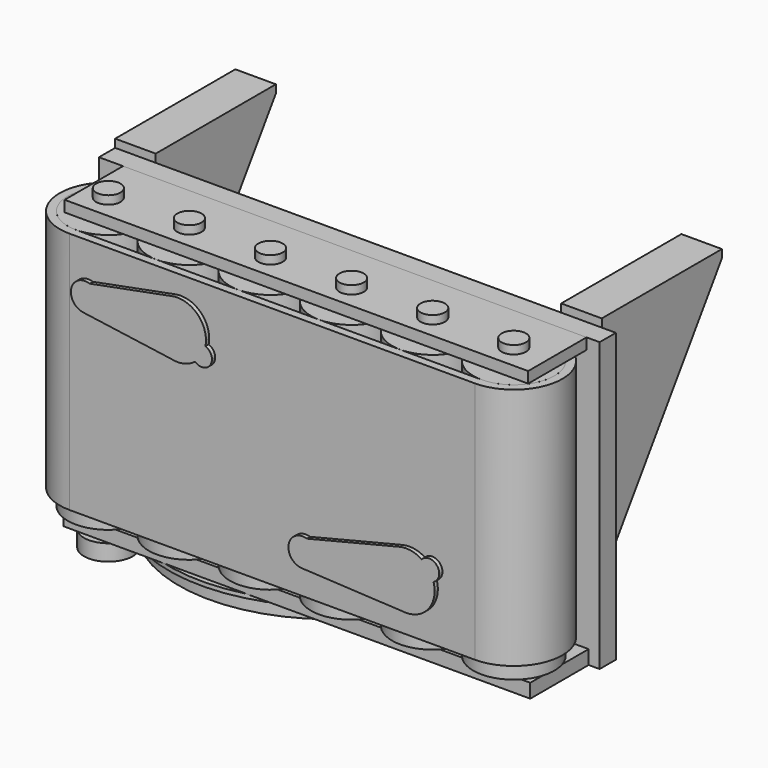
from build123d import *

# Parameters (mm, degrees)
F0_R      = 50
F1_DEPTH  = 300
F2_DEPTH  = 20
F3_R      = 15
F4_DEPTH  = 25
F5_DEPTH  = 345
F6_R      = 30
F7_DEPTH  = 20
F9_DEPTH  = 300
F10_W     = 617.369171232
F10_H     = 354.843031615
F11_DEPTH = 25
F12_W     = 571.5557485819
F12_H     = 13.6696398258
F13_DEPTH = 90
F14_W     = 575.6089426577
F14_H     = 17.266811803
F15_DEPTH = 90
F17_DEPTH = 50
F19_W     = 290.3259024024
F19_H     = 23.030102253
F20_DEPTH = 174
F22_DEPTH = 290.3259024024
F23_R     = 187.1632519627
F24_DEPTH = 20
F25_R     = 15
F26_DEPTH = 70
F28_DEPTH = 5
F29_R     = 199.2283933236
F30_DEPTH = 5
F31_R     = 2.5
F32_DEPTH = 2
F33_COUNT = 18
F34_W     = 50
F34_H     = 185.2015340328
F35_DEPTH = 10
F36_W     = 50
F36_H     = 185.2015340328
F37_DEPTH = 10
F38_R     = 10
F39_DEPTH = 60
F40_W     = 67.3258155584
F40_H     = 104.313146323
F41_DEPTH = 139


with BuildPart() as f1:
    # F0 (on Top) → F1 (new body)
    with BuildSketch(Plane.XY):
        Circle(F0_R)
    extrude(amount=F1_DEPTH)


with BuildPart() as f1b:
    # F0 (on Top) → F1, piece 2 (new body)
    with BuildSketch(Plane.XY):
        with BuildLine():
            ThreePointArc((550, 0), (500, 50), (450, 0))
            ThreePointArc((450, 0), (500, -50), (550, 0))
        make_face()
    extrude(amount=F1_DEPTH)


with BuildPart() as f1c:
    # F0 (on Top) → F1, piece 3 (new body)
    with BuildSketch(Plane.XY):
        with BuildLine():
            ThreePointArc((450, 0), (400, 50), (350, 0))
            ThreePointArc((350, 0), (400, -50), (450, 0))
        make_face()
    extrude(amount=F1_DEPTH)


with BuildPart() as f1d:
    # F0 (on Top) → F1, piece 4 (new body)
    with BuildSketch(Plane.XY):
        with BuildLine():
            ThreePointArc((350, 0), (300, 50), (250, 0))
            ThreePointArc((250, 0), (300, -50), (350, 0))
        make_face()
    extrude(amount=F1_DEPTH)


with BuildPart() as f1e:
    # F0 (on Top) → F1, piece 5 (new body)
    with BuildSketch(Plane.XY):
        with BuildLine():
            ThreePointArc((250, 0), (200, 50), (150, 0))
            ThreePointArc((150, 0), (200, -50), (250, 0))
        make_face()
    extrude(amount=F1_DEPTH)


with BuildPart() as f1f:
    # F0 (on Top) → F1, piece 6 (new body)
    with BuildSketch(Plane.XY):
        with BuildLine():
            ThreePointArc((150, 0), (100, 50), (50, 0))
            ThreePointArc((50, 0), (100, -50), (150, 0))
        make_face()
    extrude(amount=F1_DEPTH)


with BuildPart() as f2:
    # F0 (on Top) → F2 (new body)
    with BuildSketch(Plane.XY):
        Circle(F0_R)
    extrude(amount=-F2_DEPTH)


with BuildPart() as f2b:
    # F0 (on Top) → F2, piece 2 (new body)
    with BuildSketch(Plane.XY):
        with BuildLine():
            ThreePointArc((550, 0), (500, 50), (450, 0))
            ThreePointArc((450, 0), (500, -50), (550, 0))
        make_face()
    extrude(amount=-F2_DEPTH)


with BuildPart() as f2c:
    # F0 (on Top) → F2, piece 3 (new body)
    with BuildSketch(Plane.XY):
        with BuildLine():
            ThreePointArc((450, 0), (400, 50), (350, 0))
            ThreePointArc((350, 0), (400, -50), (450, 0))
        make_face()
    extrude(amount=-F2_DEPTH)


with BuildPart() as f2d:
    # F0 (on Top) → F2, piece 4 (new body)
    with BuildSketch(Plane.XY):
        with BuildLine():
            ThreePointArc((350, 0), (300, 50), (250, 0))
            ThreePointArc((250, 0), (300, -50), (350, 0))
        make_face()
    extrude(amount=-F2_DEPTH)


with BuildPart() as f2e:
    # F0 (on Top) → F2, piece 5 (new body)
    with BuildSketch(Plane.XY):
        with BuildLine():
            ThreePointArc((250, 0), (200, 50), (150, 0))
            ThreePointArc((150, 0), (200, -50), (250, 0))
        make_face()
    extrude(amount=-F2_DEPTH)


with BuildPart() as f2f:
    # F0 (on Top) → F2, piece 6 (new body)
    with BuildSketch(Plane.XY):
        with BuildLine():
            ThreePointArc((150, 0), (100, 50), (50, 0))
            ThreePointArc((50, 0), (100, -50), (150, 0))
        make_face()
    extrude(amount=-F2_DEPTH)


with BuildPart() as f4:
    # F3 (on face) → F4 (new body)
    with BuildSketch(Plane(origin=(0, 0, -20), x_dir=(1, 0, 0), z_dir=(0, 0, -1))):
        Circle(F3_R)
    extrude(amount=F4_DEPTH)


with BuildPart() as f4b:
    # F3 (on face) → F4, piece 2 (new body)
    with BuildSketch(Plane(origin=(0, 0, -20), x_dir=(1, 0, 0), z_dir=(0, 0, -1))):
        with Locations((100, 0)):
            Circle(F3_R)
    extrude(amount=F4_DEPTH)


with BuildPart() as f4c:
    # F3 (on face) → F4, piece 3 (new body)
    with BuildSketch(Plane(origin=(0, 0, -20), x_dir=(1, 0, 0), z_dir=(0, 0, -1))):
        with Locations((200, 0)):
            Circle(F3_R)
    extrude(amount=F4_DEPTH)


with BuildPart() as f4d:
    # F3 (on face) → F4, piece 4 (new body)
    with BuildSketch(Plane(origin=(0, 0, -20), x_dir=(1, 0, 0), z_dir=(0, 0, -1))):
        with Locations((300, 0)):
            Circle(F3_R)
    extrude(amount=F4_DEPTH)


with BuildPart() as f4e:
    # F3 (on face) → F4, piece 5 (new body)
    with BuildSketch(Plane(origin=(0, 0, -20), x_dir=(1, 0, 0), z_dir=(0, 0, -1))):
        with Locations((400, 0)):
            Circle(F3_R)
    extrude(amount=F4_DEPTH)


with BuildPart() as f4f:
    # F3 (on face) → F4, piece 6 (new body)
    with BuildSketch(Plane(origin=(0, 0, -20), x_dir=(1, 0, 0), z_dir=(0, 0, -1))):
        with Locations((500, 0)):
            Circle(F3_R)
    extrude(amount=F4_DEPTH)


with BuildPart() as f5:
    # F3 (on face) → F5 (new body)
    with BuildSketch(Plane(origin=(0, 0, -20), x_dir=(1, 0, 0), z_dir=(0, 0, -1))):
        Circle(F3_R)
    extrude(amount=-F5_DEPTH)


with BuildPart() as f5b:
    # F3 (on face) → F5, piece 2 (new body)
    with BuildSketch(Plane(origin=(0, 0, -20), x_dir=(1, 0, 0), z_dir=(0, 0, -1))):
        with Locations((100, 0)):
            Circle(F3_R)
    extrude(amount=-F5_DEPTH)


with BuildPart() as f5c:
    # F3 (on face) → F5, piece 3 (new body)
    with BuildSketch(Plane(origin=(0, 0, -20), x_dir=(1, 0, 0), z_dir=(0, 0, -1))):
        with Locations((200, 0)):
            Circle(F3_R)
    extrude(amount=-F5_DEPTH)


with BuildPart() as f5d:
    # F3 (on face) → F5, piece 4 (new body)
    with BuildSketch(Plane(origin=(0, 0, -20), x_dir=(1, 0, 0), z_dir=(0, 0, -1))):
        with Locations((300, 0)):
            Circle(F3_R)
    extrude(amount=-F5_DEPTH)


with BuildPart() as f5e:
    # F3 (on face) → F5, piece 5 (new body)
    with BuildSketch(Plane(origin=(0, 0, -20), x_dir=(1, 0, 0), z_dir=(0, 0, -1))):
        with Locations((400, 0)):
            Circle(F3_R)
    extrude(amount=-F5_DEPTH)


with BuildPart() as f5f:
    # F3 (on face) → F5, piece 6 (new body)
    with BuildSketch(Plane(origin=(0, 0, -20), x_dir=(1, 0, 0), z_dir=(0, 0, -1))):
        with Locations((500, 0)):
            Circle(F3_R)
    extrude(amount=-F5_DEPTH)


with BuildPart() as f7:
    # F6 (on face) → F7 (new body)
    with BuildSketch(Plane(origin=(0, 0, -45), x_dir=(1, 0, 0), z_dir=(0, 0, -1))):
        Circle(F6_R)
    extrude(amount=F7_DEPTH)


with BuildPart() as f9:
    # F8 (on face) → F9 (new body)
    with BuildSketch(Plane.XY.offset(300)):
        with BuildLine():
            Line((500, 60), (0, 60))
            ThreePointArc((0, 60), (-60, 0), (0, -60))
            Line((0, -60), (500, -60))
            ThreePointArc((500, -60), (560, 0), (500, 60))
        make_face()
        with BuildLine():
            ThreePointArc((0, -50), (-50, 0), (0, 50))
            Line((0, 50), (500, 50))
            ThreePointArc((500, 50), (550, 0), (500, -50))
            Line((500, -50), (0, -50))
        make_face(mode=Mode.SUBTRACT)
    extrude(amount=-F9_DEPTH)


with BuildPart() as f11:
    # F10 (on face) → F11 (new body)
    with BuildSketch(Plane(origin=(0, 60, 0), x_dir=(-1, 0, 0), z_dir=(0, 1, 0))):
        with Locations((-249.1421122104, 137.3082045466)):
            Rectangle(F10_W, F10_H)
    extrude(amount=F11_DEPTH)

    # F19 (on face) → F20 (join)
    with BuildSketch(Plane(origin=(0, 85, 0), x_dir=(-1, 0, 0), z_dir=(0, 1, 0))):
        with Locations((-225.6603725255, -28.5982601345)):
            Rectangle(F19_W, F19_H)
    extrude(amount=F20_DEPTH)

    # F21 (on face) → F22 (join, through all)
    with BuildSketch(Plane(origin=(80.4974213243, 0, 0), x_dir=(0, -1, 0), z_dir=(-1, 0, 0))):
        Polygon((-85, 129.8807710409), (-259, -17.083209008), (-85, -17.083209008), align=None)
    extrude(amount=-F22_DEPTH)

    # F40 (on face) → F41 (cut)
    with BuildSketch(Plane(origin=(0, 259, 0), x_dir=(-1, 0, 0), z_dir=(0, 1, 0))):
        with Locations((-145.5224826932, 35.0733641535)):
            Rectangle(F40_W, F40_H)
    extrude(amount=-F41_DEPTH, mode=Mode.SUBTRACT)


with BuildPart() as f13:
    # F12 (on face) → F13 (new body)
    with BuildSketch(Plane.XZ.offset(-60)):
        with Locations((255.916647613, 307.8949004412)):
            Rectangle(F12_W, F12_H)
    extrude(amount=F13_DEPTH)


with BuildPart() as f15:
    # F14 (on face) → F15 (new body)
    with BuildSketch(Plane.XZ.offset(-60)):
        with Locations((256.457997486, -31.4799053594)):
            Rectangle(F14_W, F14_H)
    extrude(amount=F15_DEPTH)


with BuildPart() as f17:
    # F16 (on face) → F17 (new body)
    with BuildSketch(Plane(origin=(-59.5424734056, 0, 0), x_dir=(0, -1, 0), z_dir=(-1, 0, 0))):
        Polygon((-270.2015340328, 314.7297203541), (-85, 41.2701405585), (-85, 314.7297203541), align=None)
    extrude(amount=-F17_DEPTH)


with BuildPart() as f18_1:
    # F18: copy of F17
    add(f17.part.moved(Location((550, 0, 0))))

    # F34 (on face) → F35 (join)
    with BuildSketch(Plane.XY.offset(314.7297203541)):
        with Locations((515.4575265944, 177.6007670164)):
            Rectangle(F34_W, F34_H)
    extrude(amount=F35_DEPTH)


with BuildPart() as f24:
    # F23 (on face) → F24 (new body)
    with BuildSketch(Plane(origin=(0, 0, -65), x_dir=(1, 0, 0), z_dir=(0, 0, -1))):
        with Locations((143.8672691584, -162.6717150211)):
            Circle(F23_R)
    extrude(amount=-F24_DEPTH)

    # F25 (on face) → F26 (join)
    with BuildSketch(Plane(origin=(0, 0, -65), x_dir=(1, 0, 0), z_dir=(0, 0, -1))):
        with Locations((273.0099856853, -139.8850679398)):
            Circle(F25_R)
    extrude(amount=F26_DEPTH)

    # F38 (on face) → F39 (join)
    with BuildSketch(Plane(origin=(0, 0, -65), x_dir=(1, 0, 0), z_dir=(0, 0, -1))):
        with Locations((143.8672691584, -162.6717150211)):
            Circle(F38_R)
    extrude(amount=-F39_DEPTH)


with BuildPart() as f28:
    # F27 (on face) → F28 (new body)
    with BuildSketch(Plane.XZ.offset(60)):
        with BuildLine():
            ThreePointArc((290.6598971339, 33.2716024848), (303.6093206658, 38.0614510744), (309.0558983607, 50.7486497697))
            ThreePointArc((309.0558983607, 50.7486497697), (305.6933150557, 61.0628850392), (296.8977898815, 67.4134088433))
            ThreePointArc((296.8977898815, 67.4134088433), (274.3408694475, 53.8939286949), (290.6598971339, 33.2716024848))
        make_face()
        with BuildLine():
            ThreePointArc((296.8977898815, 67.4134088433), (305.6933150557, 61.0628850392), (309.0558983607, 50.7486497697))
            ThreePointArc((309.0558983607, 50.7486497697), (303.6093206658, 38.0614510744), (290.6598971339, 33.2716024848))
            Line((290.6598971339, 33.2716024848), (415.7583559022, 26.8581408344))
            ThreePointArc((415.7583559022, 26.8581408344), (384.4237307256, 59.2215727659), (410.9251114785, 95.648585813))
            Line((410.9251114785, 95.648585813), (296.8977898815, 67.4134088433))
        make_face()
        with BuildLine():
            Line((419.3376600868, 26.6746395319), (410.9251114785, 95.648585813))
            ThreePointArc((410.9251114785, 95.648585813), (384.4237307256, 59.2215727659), (415.7583559022, 26.8581408344))
            Line((415.7583559022, 26.8581408344), (419.3376600868, 26.6746395319))
        make_face()
        with BuildLine():
            ThreePointArc((438.4152543286, 91.0182146028), (425.1510828288, 96.1884645303), (410.9251114785, 95.648585813))
            Line((410.9251114785, 95.648585813), (419.3376600868, 26.6746395319))
            ThreePointArc((419.3376600868, 26.6746395319), (444.0863974283, 36.9259021903), (454.3376600868, 61.6746395319))
            ThreePointArc((454.3376600868, 61.6746395319), (454.0044818165, 66.4924680017), (453.011290306, 71.2185709997))
            ThreePointArc((453.011290306, 71.2185709997), (437.4484346974, 75.0256635752), (438.4152543286, 91.0182146028))
        make_face()
        with BuildLine():
            Line((419.3376600868, 26.6746395319), (415.7583559022, 26.8581408344))
            ThreePointArc((415.7583559022, 26.8581408344), (417.5456576332, 26.7205449619), (419.3376600868, 26.6746395319))
        make_face()
        with BuildLine():
            ThreePointArc((460.0099761477, 82.4428991548), (452.1233251081, 94.060429502), (438.4152543286, 91.0182146028))
            ThreePointArc((438.4152543286, 91.0182146028), (447.5099761477, 82.4428991548), (453.011290306, 71.2185709997))
            ThreePointArc((453.011290306, 71.2185709997), (458.116965046, 75.8291417877), (460.0099761477, 82.4428991548))
        make_face()
        with BuildLine():
            ThreePointArc((453.011290306, 71.2185709997), (447.5099761477, 82.4428991548), (438.4152543286, 91.0182146028))
            ThreePointArc((438.4152543286, 91.0182146028), (437.4484346974, 75.0256635752), (453.011290306, 71.2185709997))
        make_face()
    extrude(amount=F28_DEPTH)


with BuildPart() as f28b:
    # F27 (on face) → F28, piece 2 (new body)
    with BuildSketch(Plane.XZ.offset(60)):
        with BuildLine():
            ThreePointArc((158.9437698468, 214.6585216105), (172.3725190643, 212.5876755669), (179.7573074196, 223.9931396009))
            ThreePointArc((179.7573074196, 223.9931396009), (177.5660202204, 231.0628242042), (171.7604369571, 235.6538353078))
            ThreePointArc((171.7604369571, 235.6538353078), (167.2573074196, 223.9931396009), (158.9437698468, 214.6585216105))
        make_face()
        with BuildLine():
            ThreePointArc((158.9437698468, 214.6585216105), (167.2573074196, 223.9931396009), (171.7604369571, 235.6538353078))
            ThreePointArc((171.7604369571, 235.6538353078), (156.5881649208, 230.5061572071), (158.9437698468, 214.6585216105))
        make_face()
        with BuildLine():
            ThreePointArc((158.9437698468, 214.6585216105), (156.5881649208, 230.5061572071), (171.7604369571, 235.6538353078))
            ThreePointArc((171.7604369571, 235.6538353078), (172.2275421578, 238.9269761977), (172.3837084229, 242.2295888984))
            ThreePointArc((172.3837084229, 242.2295888984), (159.6852716445, 269.2043971067), (130.804263973, 276.6056112211))
            ThreePointArc((130.804263973, 276.6056112211), (102.3888480283, 242.8293771651), (129.6301107961, 208.0992252344))
            Line((129.6301107961, 208.0992252344), (135.4836712828, 207.2812003967))
            ThreePointArc((135.4836712828, 207.2812003967), (147.8830110561, 208.8414975451), (158.9437698468, 214.6585216105))
        make_face()
        with BuildLine():
            ThreePointArc((129.6301107961, 208.0992252344), (132.5395926923, 207.5664306063), (135.4836712828, 207.2812003967))
            Line((135.4836712828, 207.2812003967), (129.6301107961, 208.0992252344))
        make_face()
        with BuildLine():
            ThreePointArc((129.6301107961, 208.0992252344), (102.3888480283, 242.8293771651), (130.804263973, 276.6056112211))
            Line((130.804263973, 276.6056112211), (29.1103684715, 257.1417730242))
            ThreePointArc((29.1103684715, 257.1417730242), (37.6006407713, 250.7503069973), (40.8273711056, 240.6249046326))
            ThreePointArc((40.8273711056, 240.6249046326), (34.8135364221, 227.4219501783), (20.9053132403, 223.2933254865))
            Line((20.9053132403, 223.2933254865), (129.6301107961, 208.0992252344))
        make_face()
        with BuildLine():
            ThreePointArc((40.8273711056, 240.6249046326), (37.6006407713, 250.7503069973), (29.1103684715, 257.1417730242))
            ThreePointArc((29.1103684715, 257.1417730242), (6.3199218918, 244.747606567), (20.9053132403, 223.2933254865))
            ThreePointArc((20.9053132403, 223.2933254865), (34.8135364221, 227.4219501783), (40.8273711056, 240.6249046326))
        make_face()
    extrude(amount=F28_DEPTH)


with BuildPart() as f30:
    # F29 (on face) → F30 (new body)
    with BuildSketch(Plane.XY.offset(-45)):
        with Locations((143.8672691584, 162.6717150211)):
            Circle(F29_R)
    extrude(amount=F30_DEPTH)


with BuildPart() as f32:
    # F31 (on face) → F32 (new body)
    with BuildSketch(Plane(origin=(0, 0, -45), x_dir=(1, 0, 0), z_dir=(0, 0, -1))):
        with Locations((143.3603912592, 30.6883659214)):
            Circle(F31_R)
    extrude(amount=F32_DEPTH)


with BuildPart() as f33_1:
    # F33: instance of F32
    add(f32.part.rotate(Axis((143.8672691584, 162.6717150211, -65), (0, 0, -1)), 1 * 360 / F33_COUNT))


with BuildPart() as f33_2:
    # F33: instance of F32
    add(f32.part.rotate(Axis((143.8672691584, 162.6717150211, -65), (0, 0, -1)), 2 * 360 / F33_COUNT))


with BuildPart() as f33_3:
    # F33: instance of F32
    add(f32.part.rotate(Axis((143.8672691584, 162.6717150211, -65), (0, 0, -1)), 3 * 360 / F33_COUNT))


with BuildPart() as f33_4:
    # F33: instance of F32
    add(f32.part.rotate(Axis((143.8672691584, 162.6717150211, -65), (0, 0, -1)), 4 * 360 / F33_COUNT))


with BuildPart() as f33_5:
    # F33: instance of F32
    add(f32.part.rotate(Axis((143.8672691584, 162.6717150211, -65), (0, 0, -1)), 5 * 360 / F33_COUNT))


with BuildPart() as f33_6:
    # F33: instance of F32
    add(f32.part.rotate(Axis((143.8672691584, 162.6717150211, -65), (0, 0, -1)), 6 * 360 / F33_COUNT))


with BuildPart() as f33_7:
    # F33: instance of F32
    add(f32.part.rotate(Axis((143.8672691584, 162.6717150211, -65), (0, 0, -1)), 7 * 360 / F33_COUNT))


with BuildPart() as f33_8:
    # F33: instance of F32
    add(f32.part.rotate(Axis((143.8672691584, 162.6717150211, -65), (0, 0, -1)), 8 * 360 / F33_COUNT))


with BuildPart() as f33_9:
    # F33: instance of F32
    add(f32.part.rotate(Axis((143.8672691584, 162.6717150211, -65), (0, 0, -1)), 9 * 360 / F33_COUNT))


with BuildPart() as f33_10:
    # F33: instance of F32
    add(f32.part.rotate(Axis((143.8672691584, 162.6717150211, -65), (0, 0, -1)), 10 * 360 / F33_COUNT))


with BuildPart() as f33_11:
    # F33: instance of F32
    add(f32.part.rotate(Axis((143.8672691584, 162.6717150211, -65), (0, 0, -1)), 11 * 360 / F33_COUNT))


with BuildPart() as f33_12:
    # F33: instance of F32
    add(f32.part.rotate(Axis((143.8672691584, 162.6717150211, -65), (0, 0, -1)), 12 * 360 / F33_COUNT))


with BuildPart() as f33_13:
    # F33: instance of F32
    add(f32.part.rotate(Axis((143.8672691584, 162.6717150211, -65), (0, 0, -1)), 13 * 360 / F33_COUNT))


with BuildPart() as f33_14:
    # F33: instance of F32
    add(f32.part.rotate(Axis((143.8672691584, 162.6717150211, -65), (0, 0, -1)), 14 * 360 / F33_COUNT))


with BuildPart() as f33_15:
    # F33: instance of F32
    add(f32.part.rotate(Axis((143.8672691584, 162.6717150211, -65), (0, 0, -1)), 15 * 360 / F33_COUNT))


with BuildPart() as f33_16:
    # F33: instance of F32
    add(f32.part.rotate(Axis((143.8672691584, 162.6717150211, -65), (0, 0, -1)), 16 * 360 / F33_COUNT))


with BuildPart() as f33_17:
    # F33: instance of F32
    add(f32.part.rotate(Axis((143.8672691584, 162.6717150211, -65), (0, 0, -1)), 17 * 360 / F33_COUNT))


with BuildPart() as f17_1:
    add(f17.part)

    # F36 (on face) → F37 (join)
    with BuildSketch(Plane.XY.offset(314.7297203541)):
        with Locations((-34.5424734056, 177.6007670164)):
            Rectangle(F36_W, F36_H)
    extrude(amount=F37_DEPTH)


solid = Compound([f1.part, f1b.part, f1c.part, f1d.part, f1e.part, f1f.part, f2.part, f2b.part, f2c.part, f2d.part, f2e.part, f2f.part, f4.part, f4b.part, f4c.part, f4d.part, f4e.part, f4f.part, f5.part, f5b.part, f5c.part, f5d.part, f5e.part, f5f.part, f7.part, f9.part, f11.part, f13.part, f15.part, f18_1.part, f24.part, f28.part, f28b.part, f30.part, f32.part, f33_1.part, f33_2.part, f33_3.part, f33_4.part, f33_5.part, f33_6.part, f33_7.part, f33_8.part, f33_9.part, f33_10.part, f33_11.part, f33_12.part, f33_13.part, f33_14.part, f33_15.part, f33_16.part, f33_17.part, f17_1.part])
